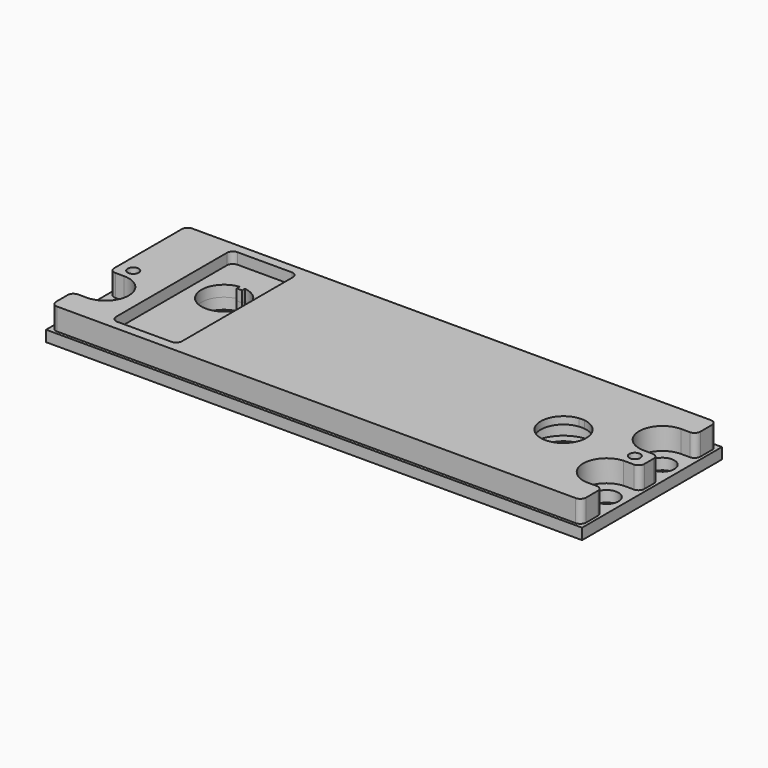
from build123d import *

# Parameters (mm, degrees)
F0_W      = 146.05
F0_H      = 47.625
F0_R      = 3.24
F0_R_2    = 1.5
F1_DEPTH  = 3
F3_DEPTH  = 25
F2_R      = 1.5
F2_W      = 18
F2_H      = 41
F4_DEPTH  = 6
F5_R      = 1.588
F6_R      = 1.5
F7_DEPTH  = 9.001
F8_R      = 8.75
F9_DEPTH  = 4
F11_DEPTH = 3


# Not quite as in the source:
# - ends of sketch curves that miss each other by under 0.0002 mm in the source are joined


with BuildPart() as f1:
    # F0 (on Top) → F1 (new body)
    with BuildSketch(Plane.XY):
        Rectangle(F0_W, F0_H)
        with Locations((-68.262, -9.5245)):
            Circle(F0_R, mode=Mode.SUBTRACT)
        with Locations((68.262, -9.5245)):
            Circle(F0_R, mode=Mode.SUBTRACT)
        with BuildLine():
            Line((72.225, -15.859485), (72.225, -23.0125))
            Line((72.225, -23.0125), (-72.225, -23.0125))
            Line((-72.225, -23.0125), (-72.225, -15.874133))
            Line((-72.225, -15.874133), (-68.193705, -15.874133))
            ThreePointArc((-68.193705, -15.874133), (-61.912367271, -9.4562050029), (-68.3302949971, -3.174867271))
            Line((-68.3302949971, -3.174867271), (-72.225, -3.174867))
            Line((-72.225, -3.174867), (-72.225, 3.1745))
            Line((-72.225, 3.1745), (-72.225, 15.8745))
            Line((-72.225, 15.8745), (-72.225, 23.0125))
            Line((-72.225, 23.0125), (72.225, 23.0125))
            Line((72.225, 23.0125), (72.225, 15.8745))
            Line((72.225, 15.8745), (68.262, 15.8745))
            ThreePointArc((68.262, 15.8745), (61.912, 9.5245), (68.262, 3.1745))
            Line((68.262, 3.1745), (72.225, 3.1745))
            Line((72.225, 3.1745), (72.225, -3.189515))
            Line((72.225, -3.189515), (67.825573, -3.189515))
            ThreePointArc((67.825573, -3.189515), (61.9270152731, -9.9609269812), (68.6984269812, -15.8594847269))
            Line((68.6984269812, -15.8594847269), (72.225, -15.859485))
        make_face(mode=Mode.SUBTRACT)
        with Locations((68.262, 9.5245)):
            Circle(F0_R, mode=Mode.SUBTRACT)
        with BuildLine():
            Line((-72.225, -23.0125), (72.225, -23.0125))
            Line((72.225, -23.0125), (72.225, -15.859485))
            Line((72.225, -15.859485), (68.698427, -15.859485))
            ThreePointArc((68.698427, -15.859485), (61.9270152731, -9.9609269812), (67.8255730188, -3.1895152731))
            Line((67.8255730188, -3.1895152731), (72.225, -3.189515))
            Line((72.225, -3.189515), (72.225, 3.1745))
            Line((72.225, 3.1745), (68.262, 3.1745))
            ThreePointArc((68.262, 3.1745), (61.912, 9.5245), (68.262, 15.8745))
            Line((68.262, 15.8745), (72.225, 15.8745))
            Line((72.225, 15.8745), (72.225, 23.0125))
            Line((72.225, 23.0125), (-72.225, 23.0125))
            Line((-72.225, 23.0125), (-72.225, 15.8745))
            Line((-72.225, 15.8745), (-72.225, 3.1745))
            Line((-72.225, 3.1745), (-72.225, -3.174867))
            Line((-72.225, -3.174867), (-68.330295, -3.174867))
            ThreePointArc((-68.330295, -3.174867), (-61.912367271, -9.4562050029), (-68.1937050029, -15.874132729))
            Line((-68.1937050029, -15.874132729), (-72.225, -15.874133))
            Line((-72.225, -15.874133), (-72.225, -23.0125))
        make_face()
        with Locations((-68.330295, 0)):
            Circle(F0_R_2, mode=Mode.SUBTRACT)
        with Locations((68.330295, 0)):
            Circle(F0_R_2, mode=Mode.SUBTRACT)
    extrude(amount=-F1_DEPTH)

    # F2 (on face) → F3 (cut)
    with BuildSketch(Plane.XY):
        with BuildLine():
            ThreePointArc((-49.662367271, 12.8544699203), (-53.0227200539, 2.0583408139), (-42.712367271, 6.7))
            ThreePointArc((-42.712367271, 6.7), (-44.2707080849, 10.8103527829), (-48.162367271, 12.8544699203))
            Line((-48.162367271, 12.8544699203), (-48.162367271, 11.9))
            Line((-48.162367271, 11.9), (-49.662367271, 11.9))
            Line((-49.662367271, 11.9), (-49.662367271, 12.8544699203))
        make_face()
        with BuildLine():
            ThreePointArc((48.16237, 6.1544699203), (44.8020172171, -4.6416591861), (55.11237, 0))
            ThreePointArc((55.11237, 0), (53.5540291861, 4.1103527829), (49.66237, 6.1544699203))
            Line((49.66237, 6.1544699203), (49.66237, 5.2))
            Line((49.66237, 5.2), (48.16237, 5.2))
            Line((48.16237, 5.2), (48.16237, 6.1544699203))
        make_face()
    extrude(amount=-F3_DEPTH, mode=Mode.SUBTRACT)

    # F6 (on face) → F7 (cut, through all)
    with BuildSketch(Plane.XY.offset(6)):
        with Locations((-68.3302949971, 0)):
            Circle(F6_R)
        with Locations((68.3302949971, 0)):
            Circle(F6_R)
    extrude(amount=-F7_DEPTH, mode=Mode.SUBTRACT)


with BuildPart() as f4:
    # F2 (on face) → F4 (new body)
    with BuildSketch(Plane.XY):
        with BuildLine():
            Line((-72.225, -15.874133), (-72.225, -23.0125))
            Line((-72.225, -23.0125), (72.225, -23.0125))
            Line((72.225, -23.0125), (72.225, -15.859485))
            Line((72.225, -15.859485), (68.698427, -15.859485))
            ThreePointArc((68.698427, -15.859485), (61.9270152731, -9.9609269812), (67.8255730188, -3.1895152731))
            Line((67.8255730188, -3.1895152731), (72.225, -3.189515))
            Line((72.225, -3.189515), (72.225, 3.1745))
            Line((72.225, 3.1745), (68.262, 3.1745))
            ThreePointArc((68.262, 3.1745), (61.912, 9.5245), (68.262, 15.8745))
            Line((68.262, 15.8745), (72.225, 15.8745))
            Line((72.225, 15.8745), (72.225, 23.0125))
            Line((72.225, 23.0125), (-72.225, 23.0125))
            Line((-72.225, 23.0125), (-72.225, 15.8745))
            Line((-72.225, 15.8745), (-72.225, 3.1745))
            Line((-72.225, 3.1745), (-72.225, -3.174867))
            Line((-72.225, -3.174867), (-68.330295, -3.174867))
            ThreePointArc((-68.330295, -3.174867), (-61.912367271, -9.4562050029), (-68.1937050029, -15.874132729))
            Line((-68.1937050029, -15.874132729), (-72.225, -15.874133))
        make_face()
        with Locations((-68.330295, 0)):
            Circle(F2_R, mode=Mode.SUBTRACT)
        with Locations((-48.912367271, 0)):
            Rectangle(F2_W, F2_H, mode=Mode.SUBTRACT)
        with BuildLine():
            ThreePointArc((49.66237, 6.1544699203), (53.5540291861, 4.1103527829), (55.11237, 0))
            ThreePointArc((55.11237, 0), (44.8020172171, -4.6416591861), (48.16237, 6.1544699203))
            Line((48.16237, 6.1544699203), (48.16237, 7.2))
            Line((48.16237, 7.2), (49.66237, 7.2))
            Line((49.66237, 7.2), (49.66237, 6.1544699203))
        make_face(mode=Mode.SUBTRACT)
        with Locations((68.330295, 0)):
            Circle(F2_R, mode=Mode.SUBTRACT)
        with BuildLine():
            ThreePointArc((48.16237, 6.1544699203), (48.91237, 6.2), (49.66237, 6.1544699203))
            Line((49.66237, 6.1544699203), (49.66237, 7.2))
            Line((49.66237, 7.2), (48.16237, 7.2))
            Line((48.16237, 7.2), (48.16237, 6.1544699203))
        make_face()
    extrude(amount=F4_DEPTH)

    # F5
    f5_edges = [f4.edges().sort_by_distance(p)[0] for p in [
        (-72.225, -23.0125, 3),
        (-72.225, -15.874133, 3),
        (-72.225, -3.174867, 3),
        (-72.225, 23.0125, 3),
        (72.225, -23.0125, 3),
        (72.225, -15.859485, 3),
        (72.225, -3.189515, 3),
        (72.225, 3.1745, 3),
        (72.225, 15.8745, 3),
        (72.225, 23.0125, 3),
        (-57.912367, 20.5, 3),
        (-39.912367, 20.5, 3),
        (-39.912367, -20.5, 3),
        (-57.912367, -20.5, 3),
    ]]
    fillet(f5_edges, radius=F5_R)

    # F8 (on face) → F9 (cut)
    with BuildSketch(Plane.XY):
        with Locations((48.91237, 0)):
            Circle(F8_R)
    extrude(amount=F9_DEPTH, mode=Mode.SUBTRACT)

    # F2 (on face) + F10 (on face) → F11 (join)
    with BuildSketch(Plane.XY):
        with Locations((-48.912367271, 0)):
            Rectangle(F2_W, F2_H)
        with BuildLine():
            ThreePointArc((-48.162367271, 12.8544699203), (-44.2707080849, 10.8103527829), (-42.712367271, 6.7))
            ThreePointArc((-42.712367271, 6.7), (-53.0227200539, 2.0583408139), (-49.662367271, 12.8544699203))
            Line((-49.662367271, 12.8544699203), (-49.662367271, 13.9))
            Line((-49.662367271, 13.9), (-48.162367271, 13.9))
            Line((-48.162367271, 13.9), (-48.162367271, 12.8544699203))
        make_face(mode=Mode.SUBTRACT)
    with BuildSketch(Plane.XY):
        with BuildLine():
            ThreePointArc((-49.662367271, 12.8544699203), (-48.912367271, 12.9), (-48.162367271, 12.8544699203))
            Line((-48.162367271, 12.8544699203), (-48.162367271, 13.9))
            Line((-48.162367271, 13.9), (-49.662367271, 13.9))
            Line((-49.662367271, 13.9), (-49.662367271, 12.8544699203))
        make_face()
        with BuildLine():
            Line((-48.162367271, 11.9), (-48.162367271, 12.8544699203))
            ThreePointArc((-48.162367271, 12.8544699203), (-48.912367271, 12.9), (-49.662367271, 12.8544699203))
            Line((-49.662367271, 12.8544699203), (-49.662367271, 11.9))
            Line((-49.662367271, 11.9), (-48.162367271, 11.9))
        make_face()
    extrude(amount=F11_DEPTH)


solid = Compound([f1.part, f4.part])
